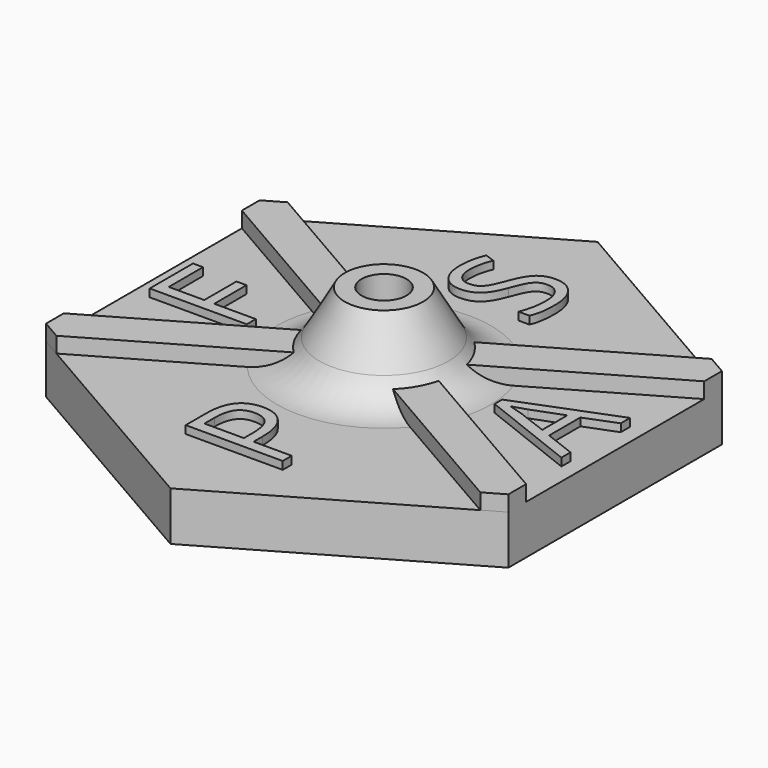
from build123d import *

# Parameters (mm, degrees)
F0_R         = 4.7625
F1_DEPTH     = 3.175
F5_DEPTH     = 1.016
F6_TEXT_SIZE = 8.8194444444
F7_DEPTH     = 0.508


# Not quite as in the source:
# - Text() gives the source's letters only with a copy of the font that has no kerning and outlines rounded to 1/6400 em; it was checked with that copy


with BuildPart() as f1:
    # F0 (on Top) → F1 (new body)
    with BuildSketch(Plane.XY):
        Polygon((15, -8.6602540378), (15, 8.6602540378), (0, 17.3205080757), (-15, 8.6602540378), (-15, -8.6602540378), (0, -17.3205080757), align=None)
        Circle(F0_R, mode=Mode.SUBTRACT)
    extrude(amount=F1_DEPTH)

    # F2 (on Front) → F3 (revolve)
    with BuildSketch(Plane.XZ):
        with BuildLine():
            Line((3.175, 0), (4.7625, 0))
            Line((4.7625, 0), (4.7625, 3.175))
            Line((4.7625, 3.175), (6.9394090512, 3.175))
            ThreePointArc((6.9394090512, 3.175), (5.3519090512, 3.600369343), (4.1897783942, 4.7625))
            Line((4.1897783942, 4.7625), (2.54, 7.62))
            Line((2.54, 7.62), (1.4605, 7.62))
            Line((1.4605, 7.62), (1.4605, 4.2545))
            Line((1.4605, 4.2545), (3.175, 2.54))
            Line((3.175, 2.54), (3.175, 0))
        make_face()
    revolve(axis=Axis((0, 0, 3.81), (0, 0, 1)))

    # F4 (on face) → F5 (join)
    with BuildSketch(Plane.XY.offset(3.175)):
        Polygon((13.7554, -9.3788241829), (15, -8.6602540378), (15, -7.2231137478), (4.0869659831, -0.9224706204), (2.8423659831, -3.0781810555), align=None)
        Polygon((15, 8.6602540378), (13.7554, 9.3788241829), (2.8423659831, 3.0781810555), (4.0869659831, 0.9224706204), (15, 7.2231137478), align=None)
        Polygon((-15, 8.6602540378), (-15, 7.2231137478), (-4.0869659831, 0.9224706204), (-2.8423659831, 3.0781810555), (-13.7554, 9.3788241829), align=None)
        Polygon((-15, -8.6602540378), (-13.7554, -9.3788241829), (-2.8423659831, -3.0781810555), (-4.0869659831, -0.9224706204), (-15, -7.2231137478), align=None)
    extrude(amount=F5_DEPTH)

    # F6 (on face) → F7 (join)
    with BuildSketch(Plane.XY.offset(3.175)):
        with Locations(Location((-7.62, -2.473578559), (0, 0, 90))):
            Text('F', F6_TEXT_SIZE, font='Open Sans', text_align=(TextAlign.LEFT, TextAlign.BOTTOM))
        with Locations(Location((3.175, 7.62), (0, 0, 90))):
            Text('S', F6_TEXT_SIZE, font='Open Sans', text_align=(TextAlign.LEFT, TextAlign.BOTTOM))
        with Locations(Location((3.175, -13.0494704861), (0, 0, 90))):
            Text('P', F6_TEXT_SIZE, font='Open Sans', text_align=(TextAlign.LEFT, TextAlign.BOTTOM))
        with Locations(Location((13.97, -3.0764702691), (0, 0, 90))):
            Text('A', F6_TEXT_SIZE, font='Open Sans', text_align=(TextAlign.LEFT, TextAlign.BOTTOM))
    extrude(amount=F7_DEPTH)


solid = f1.part
